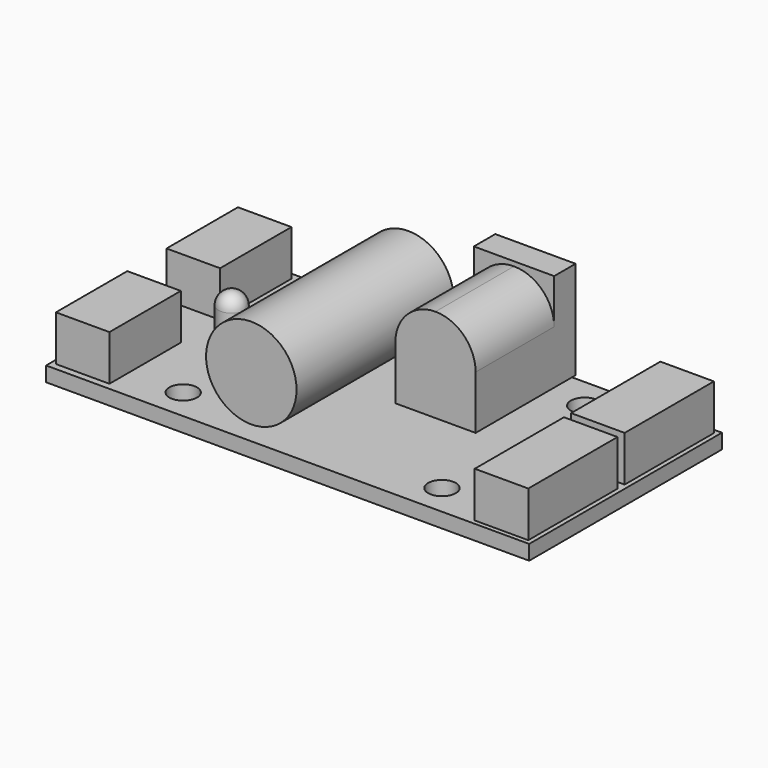
from build123d import *

# Parameters (mm, degrees)
F0_W           = 6
F0_H           = 10
F0_R           = 1.55
F0_R_2         = 1.5
F0_W_2         = 10
F0_H_2         = 22
F0_H_3         = 12.5
F0_W_3         = 9
F0_H_4         = 11
F0_H_5         = 2.5
F1_DEPTH       = 1.66
F0_H_6         = 0.5
F2_DEPTH       = 11
F3_DEPTH       = 10.5
F4_R           = 4.49999
F5_R           = 3.25
F6_DEPTH       = 10
F7_DEPTH       = 5.2
F8_R           = 1.5
F9_R           = 5.07
F10_DEPTH      = 11
F10_DEPTH_BACK = 11
F11_DEPTH      = 5.1
F12_W          = 1
F12_H          = 1
F13_DEPTH      = 2.6


# Not quite as in the source:
# - a fillet or chamfer is up to 0.001 mm smaller than in the source, because OpenCascade refuses the exact size


with BuildPart() as f1:
    # F0 (on Top) → F1 (new body)
    with BuildSketch(Plane.XY):
        Polygon((-27.07, -13.5), (27.07, -13.5), (27.07, 13.5), (10.27, 13.5), (10.27, 11), (10.27, 0), (1.27, 0), (1.27, 11), (1.27, 13.5), (-27.07, 13.5), align=None)
        with Locations((-23.57, -7.75)):
            Rectangle(F0_W, F0_H, mode=Mode.SUBTRACT)
        with Locations((-14.5, -10)):
            Circle(F0_R, mode=Mode.SUBTRACT)
        with Locations((-17.07, 0)):
            Circle(F0_R_2, mode=Mode.SUBTRACT)
        with Locations((-6.07, 0)):
            Rectangle(F0_W_2, F0_H_2, mode=Mode.SUBTRACT)
        with Locations((14.5, -10)):
            Circle(F0_R, mode=Mode.SUBTRACT)
        with Locations((23.57, -6.75)):
            Rectangle(F0_W, F0_H_3, mode=Mode.SUBTRACT)
        with Locations((-23.57, 7.75)):
            Rectangle(F0_W, F0_H, mode=Mode.SUBTRACT)
        with Locations((-14.5, 10)):
            Circle(F0_R, mode=Mode.SUBTRACT)
        with Locations((23.57, 6.75)):
            Rectangle(F0_W, F0_H_3, mode=Mode.SUBTRACT)
        with Locations((14.5, 10)):
            Circle(F0_R, mode=Mode.SUBTRACT)
        with Locations((-6.07, 0)):
            Rectangle(F0_W_2, F0_H_2)
        with Locations((5.77, 5.5)):
            Rectangle(F0_W_3, F0_H_4)
        with Locations((23.57, 6.75)):
            Rectangle(F0_W, F0_H_3)
        with Locations((23.57, -6.75)):
            Rectangle(F0_W, F0_H_3)
        with Locations((-23.57, 7.75)):
            Rectangle(F0_W, F0_H)
        with Locations((-23.57, -7.75)):
            Rectangle(F0_W, F0_H)
        with Locations((5.77, 12.25)):
            Rectangle(F0_W_3, F0_H_5)
        with Locations((-17.07, 0)):
            Circle(F0_R_2)
    extrude(amount=-F1_DEPTH)

    # F12 (on face) → F13 (join)
    with BuildSketch(Plane(origin=(0, 0, -1.66), x_dir=(1, 0, 0), z_dir=(0, 0, -1))):
        Rectangle(F12_W, F12_H)
        with Locations((0, 7)):
            Rectangle(F12_W, F12_H)
        with Locations((5.5, 7)):
            Rectangle(F12_W, F12_H)
        with Locations((11, 7)):
            Rectangle(F12_W, F12_H)
        with Locations((11, 0)):
            Rectangle(F12_W, F12_H)
        with Locations((5.5, 0)):
            Rectangle(F12_W, F12_H)
        with Locations((11, -7)):
            Rectangle(F12_W, F12_H)
        with Locations((5.5, -7)):
            Rectangle(F12_W, F12_H)
        with Locations((0, -7)):
            Rectangle(F12_W, F12_H)
        with Locations((-5.5, -7)):
            Rectangle(F12_W, F12_H)
        with Locations((-5.5, 0)):
            Rectangle(F12_W, F12_H)
        with Locations((-5.5, 7)):
            Rectangle(F12_W, F12_H)
        with Locations((-11, 7)):
            Rectangle(F12_W, F12_H)
        with Locations((-11, 0)):
            Rectangle(F12_W, F12_H)
        with Locations((-11, -7)):
            Rectangle(F12_W, F12_H)
    extrude(amount=F13_DEPTH)


with BuildPart() as f2:
    # F0 (on Top) → F2 (new body)
    with BuildSketch(Plane.XY):
        with Locations((5.77, 12.25)):
            Rectangle(F0_W_3, F0_H_5)
        with Locations((5.77, 13.75)):
            Rectangle(F0_W_3, F0_H_6)
    extrude(amount=F2_DEPTH)

    # F0 (on Top) → F3 (join)
    with BuildSketch(Plane.XY):
        with Locations((5.77, 5.5)):
            Rectangle(F0_W_3, F0_H_4)
    extrude(amount=F3_DEPTH)

    # F4 (radius 4.5 in the source; OpenCascade refuses exactly that, so slightly less here)
    f4_edges = [f2.edges().sort_by_distance(p)[0] for p in [
        (1.27, 5.5, 10.5),
        (10.27, 5.5, 10.5),
    ]]
    fillet(f4_edges, radius=F4_R)

    # F5 (on face) → F6 (cut)
    with BuildSketch(Plane(origin=(0, 14, 0), x_dir=(-1, 0, 0), z_dir=(0, 1, 0))):
        with Locations((-5.77, 6.3)):
            Circle(F5_R)
    extrude(amount=-F6_DEPTH, mode=Mode.SUBTRACT)


with BuildPart() as f7:
    # F0 (on Top) → F7 (new body)
    with BuildSketch(Plane.XY):
        with Locations((-17.07, 0)):
            Circle(F0_R_2)
    extrude(amount=F7_DEPTH)

    # F8
    f8_edges = [f7.edges().sort_by_distance(p)[0] for p in [
        (-18.57, 0, 5.2),
    ]]
    fillet(f8_edges, radius=F8_R)


with BuildPart() as f10:
    # F9 (on Front) → F10 (new body, two sides)
    with BuildSketch(Plane.XZ) as f10_sk:
        with Locations((-6.07, 5.07)):
            Circle(F9_R)
    extrude(amount=F10_DEPTH)
    extrude(f10_sk.sketch, amount=-F10_DEPTH_BACK)


with BuildPart() as f11:
    # F0 (on Top) → F11 (new body)
    with BuildSketch(Plane.XY):
        with Locations((23.57, 6.75)):
            Rectangle(F0_W, F0_H_3)
    extrude(amount=F11_DEPTH)


with BuildPart() as f11b:
    # F0 (on Top) → F11, piece 2 (new body)
    with BuildSketch(Plane.XY):
        with Locations((23.57, -6.75)):
            Rectangle(F0_W, F0_H_3)
    extrude(amount=F11_DEPTH)


with BuildPart() as f11c:
    # F0 (on Top) → F11, piece 3 (new body)
    with BuildSketch(Plane.XY):
        with Locations((-23.57, -7.75)):
            Rectangle(F0_W, F0_H)
    extrude(amount=F11_DEPTH)


with BuildPart() as f11d:
    # F0 (on Top) → F11, piece 4 (new body)
    with BuildSketch(Plane.XY):
        with Locations((-23.57, 7.75)):
            Rectangle(F0_W, F0_H)
    extrude(amount=F11_DEPTH)


solid = Compound([f1.part, f2.part, f7.part, f10.part, f11.part, f11b.part, f11c.part, f11d.part])
